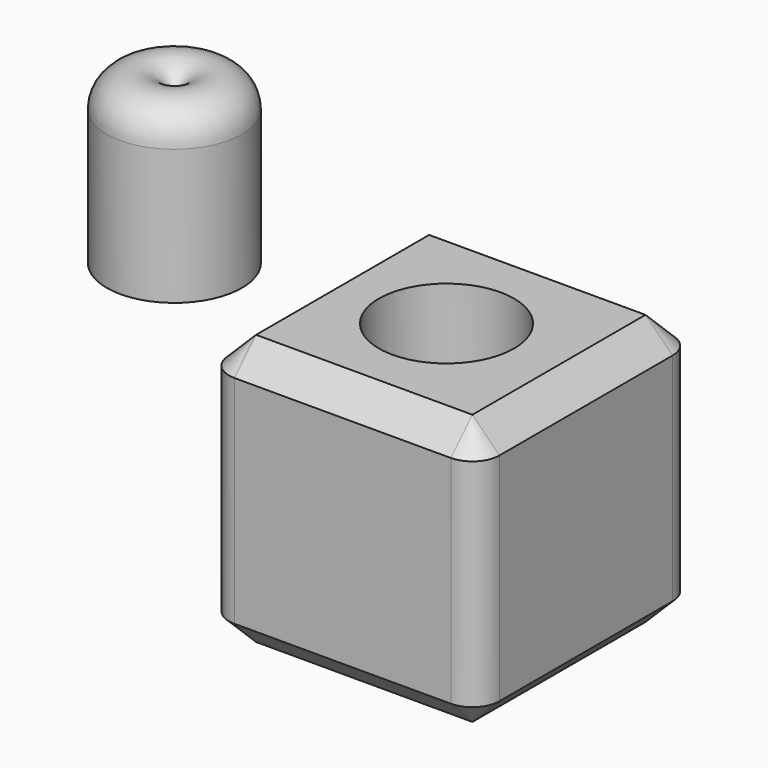
from build123d import *

# Parameters (mm, degrees)
F2_W      = 50.8
F2_H      = 50.8
F3_DEPTH  = 50.8
F4_R      = 5.08
F5_R      = 5.08
F6_R      = 5.08
F7_SIZE   = 5.07999
F8_SIZE   = 5.07999
F9_R      = 12.7
F10_DEPTH = 25.4
F11_R     = 12.6684377853
F12_DEPTH = 25.4


# Not quite as in the source:
# - a fillet or chamfer is up to 0.001 mm smaller than in the source, because OpenCascade refuses the exact size


with BuildPart() as f1:
    # F0 (on Front) → F1 (revolve)
    with BuildSketch(Plane.XZ):
        with BuildLine():
            ThreePointArc((-27.421294558, 35.2369621396), (-33.9731451561, 41.1732071319), (-40.121294558, 34.8197820872))
            Line((-40.121294558, 34.8197820872), (-40.121294558, 9.4197820872))
            Line((-40.121294558, 9.4197820872), (-27.421294558, 9.4197820872))
            Line((-27.421294558, 9.4197820872), (-27.421294558, 35.2369621396))
        make_face()
    revolve(axis=Axis((-27.421294558, 0, 22.3283721134), (0, 0, 1)))


with BuildPart() as f3:
    # F2 (on Front) → F3 (new body)
    with BuildSketch(Plane.XZ):
        with Locations((44.8210335612, 7.6070784867)):
            Rectangle(F2_W, F2_H)
    extrude(amount=F3_DEPTH)

    # F4
    f4_edges = [f3.edges().sort_by_distance(p)[0] for p in [
        (19.421034, -50.8, 7.607078),
    ]]
    fillet(f4_edges, radius=F4_R)

    # F5
    f5_edges = [f3.edges().sort_by_distance(p)[0] for p in [
        (70.221034, -50.8, 7.607078),
        (70.221034, 0, 7.607078),
    ]]
    fillet(f5_edges, radius=F5_R)

    # F6
    f6_edges = [f3.edges().sort_by_distance(p)[0] for p in [
        (19.421034, 0, 7.607078),
    ]]
    fillet(f6_edges, radius=F6_R)

    # F7 (size 5.08 in the source; OpenCascade refuses exactly that, so slightly less here)
    f7_edges = [f3.edges().sort_by_distance(p)[0] for p in [
        (44.821034, 0, 33.007078),
        (20.908931, -1.487898, 33.007078),
        (68.733136, -1.487898, 33.007078),
        (19.421034, -25.4, 33.007078),
        (70.221034, -25.4, 33.007078),
        (20.908931, -49.312102, 33.007078),
        (68.733136, -49.312102, 33.007078),
        (44.821034, -50.8, 33.007078),
    ]]
    chamfer(f7_edges, length=F7_SIZE)

    # F8 (size 5.08 in the source; OpenCascade refuses exactly that, so slightly less here)
    f8_edges = [f3.edges().sort_by_distance(p)[0] for p in [
        (44.821034, 0, -17.792922),
        (20.908931, -1.487898, -17.792922),
        (68.733136, -1.487898, -17.792922),
        (19.421034, -25.4, -17.792922),
        (70.221034, -25.4, -17.792922),
        (20.908931, -49.312102, -17.792922),
        (68.733136, -49.312102, -17.792922),
        (44.821034, -50.8, -17.792922),
    ]]
    chamfer(f8_edges, length=F8_SIZE)

    # F9 (on face) → F10 (cut)
    with BuildSketch(Plane.XY.offset(33.0070784867)):
        with Locations((44.0752767026, -25.4682991654)):
            Circle(F9_R)
    extrude(amount=-F10_DEPTH, mode=Mode.SUBTRACT)

    # F11 (on face) → F12 (cut)
    with BuildSketch(Plane.XY.offset(7.6070784867)):
        with Locations((44.0752767026, -25.4682991654)):
            Circle(F11_R)
    extrude(amount=-F12_DEPTH, mode=Mode.SUBTRACT)


solid = Compound([f1.part, f3.part])
